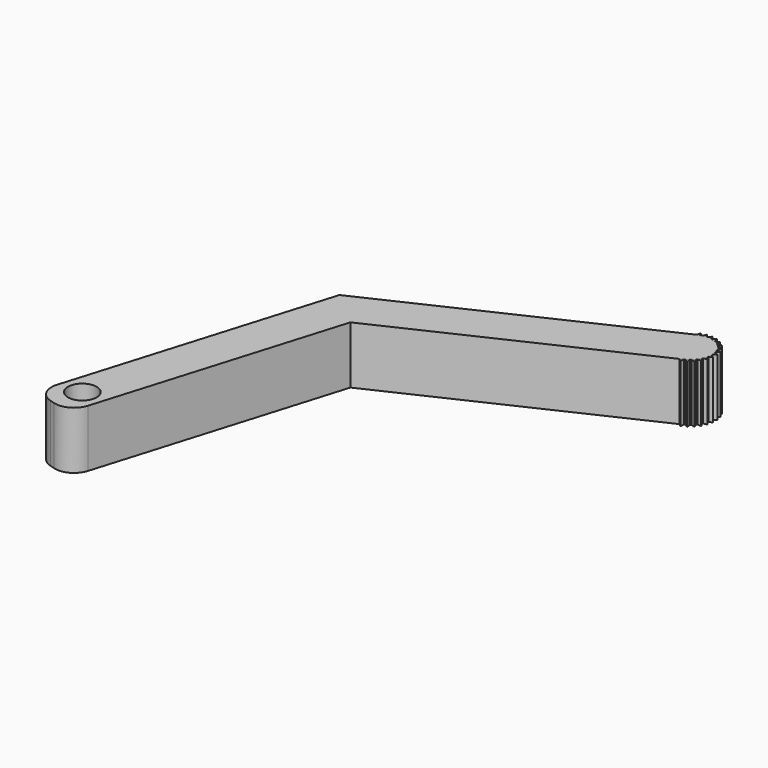
from build123d import *

# Parameters (mm, degrees)
F1_DEPTH = 7.62
F3_DEPTH = 2.54
F5_COUNT = 15
F5_ANGLE = 180
F6_DEPTH = 2.54
F7_R     = 2.54


with BuildPart() as f1:
    # F0 (on Top) → F1 (new body)
    with BuildSketch(Plane.XY):
        with BuildLine():
            Line((11.0146695097, 36.4731004384), (0, 0))
            Line((0, 0), (2.7266272251, -0.8234259605))
            Line((2.7266272251, -0.8234259605), (5.4532544502, -1.646851921))
            Line((5.4532544502, -1.646851921), (15.7336126593, 32.3947084882))
            Line((15.7336126593, 32.3947084882), (47.9269573, 47.4977598634))
            ThreePointArc((47.9269573, 47.4977598634), (44.1386573668, 48.8666412643), (45.5075387677, 52.6549411976))
            Line((45.5075387677, 52.6549411976), (11.0146695097, 36.4731004384))
        make_face()
        with BuildLine():
            ThreePointArc((5.7230184328, 2.8269117268), (4.9558837312, 1.2990741822), (3.272322829, 1.0017428832))
            ThreePointArc((3.272322829, 1.0017428832), (2.6801531345, 4.3547492715), (5.7230184328, 2.8269117268))
        make_face(mode=Mode.SUBTRACT)
        with BuildLine():
            Line((47.9269573, 47.4977598634), (45.5075387677, 52.6549411976))
            ThreePointArc((45.5075387677, 52.6549411976), (44.1386573668, 48.8666412643), (47.9269573, 47.4977598634))
        make_face()
        with BuildLine():
            Line((45.9848520759, 52.8288262339), (45.5075387677, 52.6549411976))
            Line((45.5075387677, 52.6549411976), (47.9269573, 47.4977598634))
            ThreePointArc((47.9269573, 47.4977598634), (49.1212114682, 48.548775281), (49.5654977309, 50.0763505305))
            ThreePointArc((49.5654977309, 50.0763505305), (48.4531166596, 52.3345105007), (45.9848520759, 52.8288262339))
        make_face()
    extrude(amount=F1_DEPTH)

    # F2 (on face) → F3 (join)
    with BuildSketch(Plane.XY.offset(7.62)):
        with BuildLine():
            Line((45.9848520759, 52.8288262339), (45.5075387677, 52.6549411976))
            Line((45.5075387677, 52.6549411976), (47.9269573, 47.4977598634))
            ThreePointArc((47.9269573, 47.4977598634), (49.3934438712, 51.0512875423), (45.9848520759, 52.8288262339))
        make_face()
    extrude(amount=F3_DEPTH)

    # F6 (cut): a face of the model
    f6_faces = [f1.faces().sort_by_distance(p)[0] for p in [
        (47.8122597318, 50.5891162823, 10.16),
    ]]
    extrude(f6_faces, amount=-F6_DEPTH, mode=Mode.SUBTRACT)

    # F7
    f7_edges = [f1.edges().sort_by_distance(p)[0] for p in [
        (5.453254, -1.646852, 3.81),
        (0, 0, 3.81),
    ]]
    fillet(f7_edges, radius=F7_R)


with BuildPart() as f1b:
    # F0 (on Top) → F1, piece 2 (new body)
    with BuildSketch(Plane.XY):
        with BuildLine():
            Line((45.595606563, 53.1552491662), (45.5075387677, 52.6549411976))
            ThreePointArc((45.5075387677, 52.6549411976), (45.7423110221, 52.7525463679), (45.9848520759, 52.8288262339))
            Line((45.9848520759, 52.8288262339), (45.595606563, 53.1552491662))
        make_face()
    extrude(amount=F1_DEPTH)


with BuildPart() as f5_1:
    # F5: instance of F1b
    add(f1b.part.rotate(Axis((46.7172480338, 50.0763505305, 8.89), (0, 0, -1)), 1 * F5_ANGLE / (F5_COUNT - 1)))


with BuildPart() as f5_2:
    # F5: instance of F1b
    add(f1b.part.rotate(Axis((46.7172480338, 50.0763505305, 8.89), (0, 0, -1)), 2 * F5_ANGLE / (F5_COUNT - 1)))


with BuildPart() as f5_3:
    # F5: instance of F1b
    add(f1b.part.rotate(Axis((46.7172480338, 50.0763505305, 8.89), (0, 0, -1)), 3 * F5_ANGLE / (F5_COUNT - 1)))


with BuildPart() as f5_4:
    # F5: instance of F1b
    add(f1b.part.rotate(Axis((46.7172480338, 50.0763505305, 8.89), (0, 0, -1)), 4 * F5_ANGLE / (F5_COUNT - 1)))


with BuildPart() as f5_5:
    # F5: instance of F1b
    add(f1b.part.rotate(Axis((46.7172480338, 50.0763505305, 8.89), (0, 0, -1)), 5 * F5_ANGLE / (F5_COUNT - 1)))


with BuildPart() as f5_6:
    # F5: instance of F1b
    add(f1b.part.rotate(Axis((46.7172480338, 50.0763505305, 8.89), (0, 0, -1)), 6 * F5_ANGLE / (F5_COUNT - 1)))


with BuildPart() as f5_7:
    # F5: instance of F1b
    add(f1b.part.rotate(Axis((46.7172480338, 50.0763505305, 8.89), (0, 0, -1)), 7 * F5_ANGLE / (F5_COUNT - 1)))


with BuildPart() as f5_8:
    # F5: instance of F1b
    add(f1b.part.rotate(Axis((46.7172480338, 50.0763505305, 8.89), (0, 0, -1)), 8 * F5_ANGLE / (F5_COUNT - 1)))


with BuildPart() as f5_9:
    # F5: instance of F1b
    add(f1b.part.rotate(Axis((46.7172480338, 50.0763505305, 8.89), (0, 0, -1)), 9 * F5_ANGLE / (F5_COUNT - 1)))


with BuildPart() as f5_10:
    # F5: instance of F1b
    add(f1b.part.rotate(Axis((46.7172480338, 50.0763505305, 8.89), (0, 0, -1)), 10 * F5_ANGLE / (F5_COUNT - 1)))


with BuildPart() as f5_11:
    # F5: instance of F1b
    add(f1b.part.rotate(Axis((46.7172480338, 50.0763505305, 8.89), (0, 0, -1)), 11 * F5_ANGLE / (F5_COUNT - 1)))


with BuildPart() as f5_12:
    # F5: instance of F1b
    add(f1b.part.rotate(Axis((46.7172480338, 50.0763505305, 8.89), (0, 0, -1)), 12 * F5_ANGLE / (F5_COUNT - 1)))


with BuildPart() as f5_13:
    # F5: instance of F1b
    add(f1b.part.rotate(Axis((46.7172480338, 50.0763505305, 8.89), (0, 0, -1)), 13 * F5_ANGLE / (F5_COUNT - 1)))


with BuildPart() as f5_14:
    # F5: instance of F1b
    add(f1b.part.rotate(Axis((46.7172480338, 50.0763505305, 8.89), (0, 0, -1)), 14 * F5_ANGLE / (F5_COUNT - 1)))


solid = Compound([f1.part, f1b.part, f5_1.part, f5_2.part, f5_3.part, f5_4.part, f5_5.part, f5_6.part, f5_7.part, f5_8.part, f5_9.part, f5_10.part, f5_11.part, f5_12.part, f5_13.part, f5_14.part])
